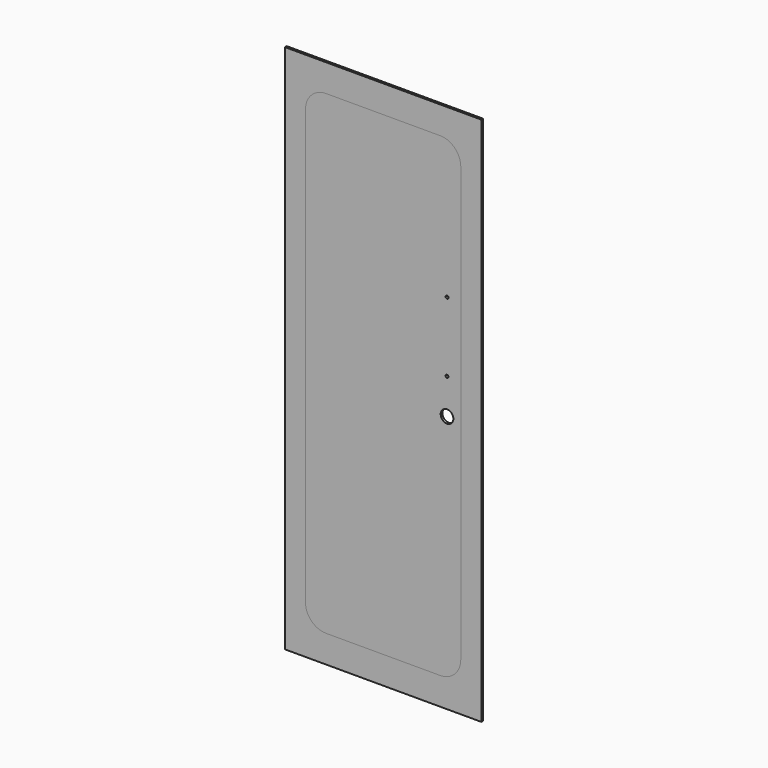
from build123d import *

# Parameters (mm, degrees)
F0_W     = 286
F0_H     = 771.5
F1_DEPTH = 3.175
F0_R     = 9.25
F0_R_2   = 2.1
F2_DEPTH = 3.175


# Not quite as in the source:
# - a length typed as a fraction of an inch, garbled in the dataset ("3 / 203.2 mm" for 3/8 in), is restored


with BuildPart() as f1:
    # F0 (on Front) → F1 (new body)
    with BuildSketch(Plane.XZ):
        with Locations((143, 385.75)):
            Rectangle(F0_W, F0_H)
        with BuildLine():
            ThreePointArc((30, 701.5), (38.7867965644, 722.7132034356), (60, 731.5))
            Line((60, 731.5), (226, 731.5))
            ThreePointArc((226, 731.5), (247.2132034356, 722.7132034356), (256, 701.5))
            Line((256, 701.5), (256, 70))
            ThreePointArc((256, 70), (247.2132034356, 48.7867965644), (226, 40))
            Line((226, 40), (60, 40))
            ThreePointArc((60, 40), (38.7867965644, 48.7867965644), (30, 70))
            Line((30, 70), (30, 701.5))
        make_face(mode=Mode.SUBTRACT)
    extrude(amount=F1_DEPTH)


with BuildPart() as f2:
    # F0 (on Front) → F2 (new body)
    with BuildSketch(Plane.XZ):
        with BuildLine():
            Line((226, 731.5), (60, 731.5))
            ThreePointArc((60, 731.5), (38.7867965644, 722.7132034356), (30, 701.5))
            Line((30, 701.5), (30, 70))
            ThreePointArc((30, 70), (38.7867965644, 48.7867965644), (60, 40))
            Line((60, 40), (226, 40))
            ThreePointArc((226, 40), (247.2132034356, 48.7867965644), (256, 70))
            Line((256, 70), (256, 701.5))
            ThreePointArc((256, 701.5), (247.2132034356, 722.7132034356), (226, 731.5))
        make_face()
        with Locations((236, 375.025)):
            Circle(F0_R, mode=Mode.SUBTRACT)
        with Locations((236, 426.375)):
            Circle(F0_R_2, mode=Mode.SUBTRACT)
        with Locations((236, 527.975)):
            Circle(F0_R_2, mode=Mode.SUBTRACT)
    extrude(amount=F2_DEPTH)


solid = Compound([f1.part, f2.part])
